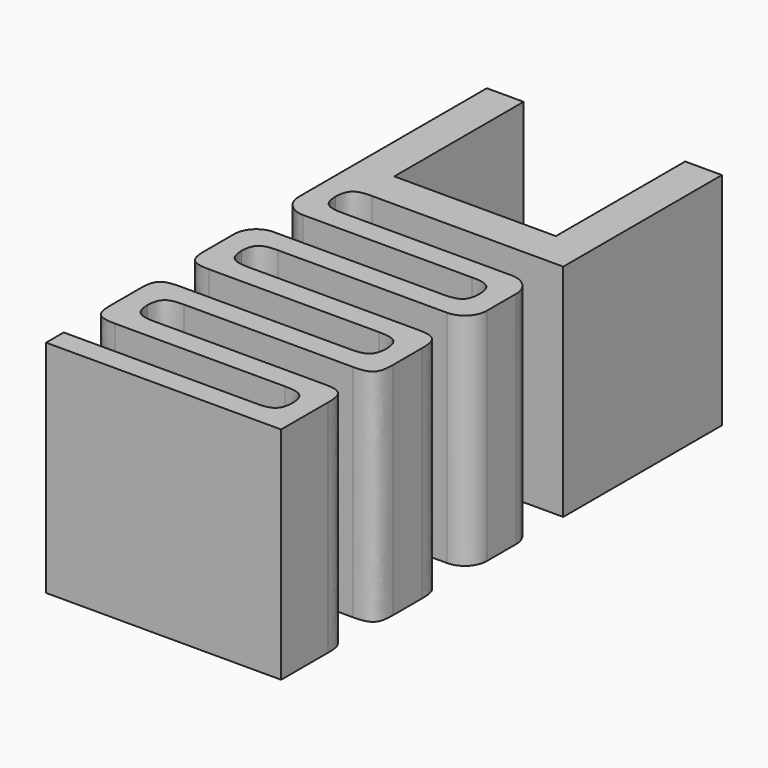
from build123d import *

# Parameters (mm, degrees)
F0_W        = 5
F0_H        = 22
F0_W_2      = 3
F0_H_2      = 5
F0_W_3      = 2.8575498313
F1_DEPTH    = 30
F2_T1_DEPTH = 30
F2_T3_DEPTH = 45


# Not quite as in the source:
# - a fillet or chamfer that OpenCascade refuses, or shapes differently, is made with other operations: its cross-section is extruded or revolved along the edge and cut away or added


with BuildPart() as f1:
    # F0 (on Top) → F1 (new body)
    with BuildSketch(Plane.XY):
        with Locations((-16.665090844, -16.7530454993)):
            Rectangle(F0_W, F0_H)
        Polygon((7.834909156, -27.7530454993), (-14.165090844, -27.7530454993), (-19.165090844, -27.7530454993), (-19.165090844, -32.7530454993), (-16.165090844, -32.7530454993), (12.834909156, -32.7530454993), (12.834909156, -27.7530454993), align=None)
        with Locations((10.334909156, -16.7530454993)):
            Rectangle(F0_W, F0_H)
        with Locations((-17.665090844, -35.2530454993)):
            Rectangle(F0_W_2, F0_H_2)
        with BuildLine():
            Line((-16.165090844, -37.7530454993), (-19.165090844, -37.7530454993))
            ThreePointArc((-19.165090844, -37.7530454993), (-18.2864111876, -39.8743658429), (-16.165090844, -40.7530454993))
            Line((-16.165090844, -40.7530454993), (9.834909156, -40.7530454993))
            Line((9.834909156, -40.7530454993), (12.834909156, -40.7530454993))
            ThreePointArc((12.834909156, -40.7530454993), (11.9562294995, -38.6317251558), (9.834909156, -37.7530454993))
            Line((9.834909156, -37.7530454993), (-16.165090844, -37.7530454993))
        make_face()
        with Locations((11.334909156, -43.2530454993)):
            Rectangle(F0_W_2, F0_H_2)
        with BuildLine():
            Line((12.834909156, -45.7530454993), (9.834909156, -45.7530454993))
            Line((9.834909156, -45.7530454993), (-16.165090844, -45.7530454993))
            ThreePointArc((-16.165090844, -45.7530454993), (-18.2864111876, -46.6317251558), (-19.165090844, -48.7530454993))
            Line((-19.165090844, -48.7530454993), (-16.165090844, -48.7530454993))
            Line((-16.165090844, -48.7530454993), (9.834909156, -48.7530454993))
            ThreePointArc((9.834909156, -48.7530454993), (11.9562294995, -47.8743658429), (12.834909156, -45.7530454993))
        make_face()
        with Locations((-17.665090844, -51.2530454993)):
            Rectangle(F0_W_2, F0_H_2)
        Polygon((-16.165090844, -53.7530454993), (-19.165090844, -53.7530454993), (-19.165090844, -56.7530454993), (9.9773593247, -56.7530454993), (12.834909156, -56.7530454993), (12.834909156, -53.7530454993), align=None)
        with Locations((11.4061342403, -59.2530454993)):
            Rectangle(F0_W_3, F0_H_2)
        Polygon((12.834909156, -61.7530454993), (9.9773593247, -61.7530454993), (-19.165090844, -61.7530454993), (-19.165090844, -64.7530454993), (-16.165090844, -64.7530454993), (12.834909156, -64.7530454993), align=None)
        with Locations((-17.665090844, -67.2530454993)):
            Rectangle(F0_W_2, F0_H_2)
        Polygon((-16.165090844, -69.7530454993), (-19.165090844, -69.7530454993), (-19.165090844, -72.7530454993), (9.9773593247, -72.7530454993), (12.834909156, -72.7530454993), (12.834909156, -69.7530454993), align=None)
        with Locations((11.4061342403, -75.2530454993)):
            Rectangle(F0_W_3, F0_H_2)
        Polygon((12.834909156, -77.7530454993), (9.9773593247, -77.7530454993), (-19.165090844, -77.7530454993), (-19.165090844, -80.7530454993), (12.834909156, -80.7530454993), align=None)
    extrude(amount=F1_DEPTH)

    # F2: fillet of radius 3 on 18 edges, made by hand

    # F2_s2 → F2_t1 (join)
    with BuildSketch(Plane.XY):
        with BuildLine():
            add(Edge.make_bspline(
                [(-13.165090844, -37.7530454993), (-16.165090844, -37.7530454993), (-16.165090844, -34.7530454993)],
                knots=[0, 0, 0, 1, 1, 1], degree=2, weights=[1, 1.5, 1]))
            Line((-16.165090844, -34.7530454993), (-16.165090844, -37.7530454993))
            Line((-16.165090844, -37.7530454993), (-13.165090844, -37.7530454993))
        make_face()
        with BuildLine():
            add(Edge.make_bspline(
                [(-16.165090844, -35.7530454993), (-16.165090844, -32.7530454993), (-13.165090844, -32.7530454993)],
                knots=[0, 0, 0, 1, 1, 1], degree=2, weights=[1, 1.5, 1]))
            Line((-13.165090844, -32.7530454993), (-16.165090844, -32.7530454993))
            Line((-16.165090844, -32.7530454993), (-16.165090844, -35.7530454993))
        make_face()
        with BuildLine():
            add(Edge.make_bspline(
                [(6.834909156, -40.7530454993), (9.834909156, -40.7530454993), (9.834909156, -43.7530454993)],
                knots=[0, 0, 0, 1, 1, 1], degree=2, weights=[1, 1.5, 1]))
            Line((9.834909156, -43.7530454993), (9.834909156, -40.7530454993))
            Line((9.834909156, -40.7530454993), (6.834909156, -40.7530454993))
        make_face()
        with BuildLine():
            add(Edge.make_bspline(
                [(9.834909156, -42.7530454993), (9.834909156, -45.7530454993), (6.834909156, -45.7530454993)],
                knots=[0, 0, 0, 1, 1, 1], degree=2, weights=[1, 1.5, 1]))
            Line((6.834909156, -45.7530454993), (9.834909156, -45.7530454993))
            Line((9.834909156, -45.7530454993), (9.834909156, -42.7530454993))
        make_face()
        with BuildLine():
            add(Edge.make_bspline(
                [(-16.165090844, -51.7530454993), (-16.165090844, -48.7530454993), (-13.165090844, -48.7530454993)],
                knots=[0, 0, 0, 1, 1, 1], degree=2, weights=[1, 1.5, 1]))
            Line((-13.165090844, -48.7530454993), (-16.165090844, -48.7530454993))
            Line((-16.165090844, -48.7530454993), (-16.165090844, -51.7530454993))
        make_face()
        with BuildLine():
            add(Edge.make_bspline(
                [(-13.165090844, -53.7530454993), (-16.165090844, -53.7530454993), (-16.165090844, -50.7530454993)],
                knots=[0, 0, 0, 1, 1, 1], degree=2, weights=[1, 1.5, 1]))
            Line((-16.165090844, -50.7530454993), (-16.165090844, -53.7530454993))
            Line((-16.165090844, -53.7530454993), (-13.165090844, -53.7530454993))
        make_face()
        with BuildLine():
            add(Edge.make_bspline(
                [(6.9773593247, -72.7530454993), (9.9773593247, -72.7530454993), (9.9773593247, -75.7530454993)],
                knots=[0, 0, 0, 1, 1, 1], degree=2, weights=[1, 1.5, 1]))
            Line((9.9773593247, -75.7530454993), (9.9773593247, -72.7530454993))
            Line((9.9773593247, -72.7530454993), (6.9773593247, -72.7530454993))
        make_face()
        with BuildLine():
            add(Edge.make_bspline(
                [(9.9773593247, -74.7530454993), (9.9773593247, -77.7530454993), (6.9773593247, -77.7530454993)],
                knots=[0, 0, 0, 1, 1, 1], degree=2, weights=[1, 1.5, 1]))
            Line((6.9773593247, -77.7530454993), (9.9773593247, -77.7530454993))
            Line((9.9773593247, -77.7530454993), (9.9773593247, -74.7530454993))
        make_face()
        with BuildLine():
            add(Edge.make_bspline(
                [(6.9773593247, -56.7530454993), (9.9773593247, -56.7530454993), (9.9773593247, -59.7530454993)],
                knots=[0, 0, 0, 1, 1, 1], degree=2, weights=[1, 1.5, 1]))
            Line((9.9773593247, -59.7530454993), (9.9773593247, -56.7530454993))
            Line((9.9773593247, -56.7530454993), (6.9773593247, -56.7530454993))
        make_face()
        with BuildLine():
            add(Edge.make_bspline(
                [(9.9773593247, -58.7530454993), (9.9773593247, -61.7530454993), (6.9773593247, -61.7530454993)],
                knots=[0, 0, 0, 1, 1, 1], degree=2, weights=[1, 1.5, 1]))
            Line((6.9773593247, -61.7530454993), (9.9773593247, -61.7530454993))
            Line((9.9773593247, -61.7530454993), (9.9773593247, -58.7530454993))
        make_face()
        with BuildLine():
            add(Edge.make_bspline(
                [(-16.165090844, -67.7530454993), (-16.165090844, -64.7530454993), (-13.165090844, -64.7530454993)],
                knots=[0, 0, 0, 1, 1, 1], degree=2, weights=[1, 1.5, 1]))
            Line((-13.165090844, -64.7530454993), (-16.165090844, -64.7530454993))
            Line((-16.165090844, -64.7530454993), (-16.165090844, -67.7530454993))
        make_face()
        with BuildLine():
            add(Edge.make_bspline(
                [(-13.165090844, -69.7530454993), (-16.165090844, -69.7530454993), (-16.165090844, -66.7530454993)],
                knots=[0, 0, 0, 1, 1, 1], degree=2, weights=[1, 1.5, 1]))
            Line((-16.165090844, -66.7530454993), (-16.165090844, -69.7530454993))
            Line((-16.165090844, -69.7530454993), (-13.165090844, -69.7530454993))
        make_face()
    extrude(amount=F2_T1_DEPTH)

    # F2_s4 → F2_t3 (cut)
    with BuildSketch(Plane.XY.offset(-7.5)):
        with BuildLine():
            add(Edge.make_bspline(
                [(12.834909156, -56.7530454993), (12.834909156, -53.7530454993), (9.834909156, -53.7530454993)],
                knots=[0, 0, 0, 1, 1, 1], degree=2, weights=[1, 1.5, 1]))
            Line((9.834909156, -53.7530454993), (12.834909156, -53.7530454993))
            Line((12.834909156, -53.7530454993), (12.834909156, -56.7530454993))
        make_face()
        with BuildLine():
            add(Edge.make_bspline(
                [(9.834909156, -64.7530454993), (12.834909156, -64.7530454993), (12.834909156, -61.7530454993)],
                knots=[0, 0, 0, 1, 1, 1], degree=2, weights=[1, 1.5, 1]))
            Line((12.834909156, -61.7530454993), (12.834909156, -64.7530454993))
            Line((12.834909156, -64.7530454993), (9.834909156, -64.7530454993))
        make_face()
        with BuildLine():
            add(Edge.make_bspline(
                [(12.834909156, -72.7530454993), (12.834909156, -69.7530454993), (9.834909156, -69.7530454993)],
                knots=[0, 0, 0, 1, 1, 1], degree=2, weights=[1, 1.5, 1]))
            Line((9.834909156, -69.7530454993), (12.834909156, -69.7530454993))
            Line((12.834909156, -69.7530454993), (12.834909156, -72.7530454993))
        make_face()
        with BuildLine():
            add(Edge.make_bspline(
                [(-19.165090844, -69.7530454993), (-19.165090844, -72.7530454993), (-16.165090844, -72.7530454993)],
                knots=[0, 0, 0, 1, 1, 1], degree=2, weights=[1, 1.5, 1]))
            Line((-16.165090844, -72.7530454993), (-19.165090844, -72.7530454993))
            Line((-19.165090844, -72.7530454993), (-19.165090844, -69.7530454993))
        make_face()
        with BuildLine():
            add(Edge.make_bspline(
                [(-16.165090844, -61.7530454993), (-19.165090844, -61.7530454993), (-19.165090844, -64.7530454993)],
                knots=[0, 0, 0, 1, 1, 1], degree=2, weights=[1, 1.5, 1]))
            Line((-19.165090844, -64.7530454993), (-19.165090844, -61.7530454993))
            Line((-19.165090844, -61.7530454993), (-16.165090844, -61.7530454993))
        make_face()
        with BuildLine():
            add(Edge.make_bspline(
                [(-19.165090844, -53.7530454993), (-19.165090844, -56.7530454993), (-16.165090844, -56.7530454993)],
                knots=[0, 0, 0, 1, 1, 1], degree=2, weights=[1, 1.5, 1]))
            Line((-16.165090844, -56.7530454993), (-19.165090844, -56.7530454993))
            Line((-19.165090844, -56.7530454993), (-19.165090844, -53.7530454993))
        make_face()
    extrude(amount=F2_T3_DEPTH, mode=Mode.SUBTRACT)


solid = f1.part
